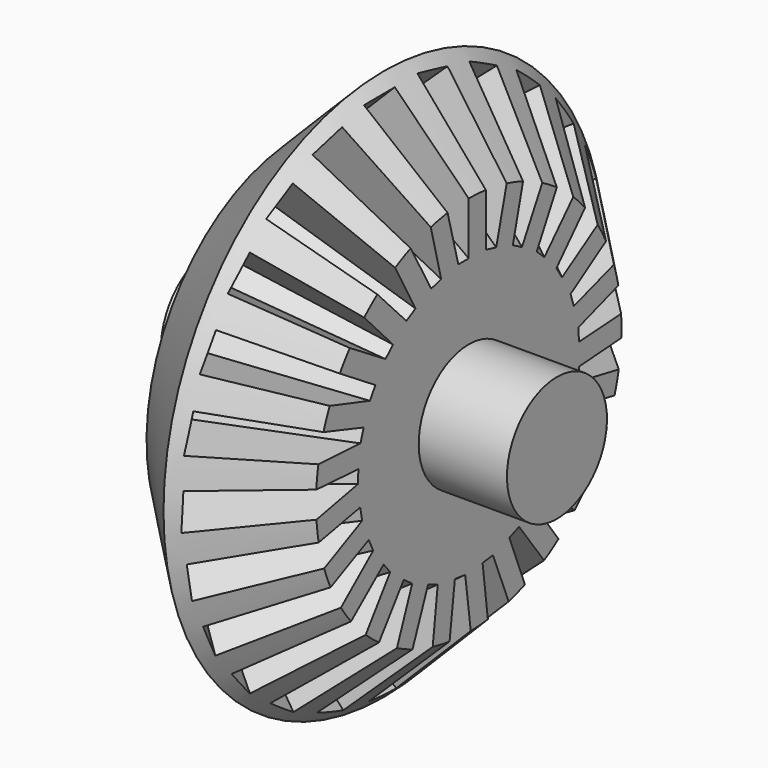
from build123d import *

# Parameters (mm, degrees)
F7_COUNT = 25
F7_ANGLE = 345.6


with BuildPart() as f1:
    # F0 (on Front) → F1 (revolve)
    with BuildSketch(Plane.XZ):
        Polygon((5.5470483679, 18.0012998082), (0.0122273423, 12.4664593884), (-0.0058063755, 4.0821318731), (-5.763291413, 4.0821318731), (-5.763291413, 0), (0, 0), (16.8451661991, 0), (16.8451661991, 4.0821318731), (11.0818887877, 4.0821318731), (11.0818887877, 12.4664787826), align=None)
    revolve(axis=Axis((8.4225830996, 0, 0), (-1, 0, 0)))


with BuildPart() as f6:
    # F5 (on face) → F6 section 0
    with BuildSketch(Plane(origin=(-5.5200079815, 0, 5.5199886393), x_dir=(0, -1, 0), z_dir=(-0.70710802, 0, 0.7071055423)), mode=Mode.PRIVATE) as f6_s0:
        Polygon((0, 16.6512121101), (0, 12.7288497215), (1.3675010996, 12.7288497215), (2.4401100818, 16.6512121101), align=None)
    loft([f6_s0.sketch, Vertex(23.5484112532, 0, 0)])


with BuildPart() as f7_1:
    # F7: instance of F6
    add(f6.part.rotate(Axis((16.8451661991, 0, 0), (-1, 0, 0)), 1 * F7_ANGLE / (F7_COUNT - 1)))


with BuildPart() as f7_2:
    # F7: instance of F6
    add(f6.part.rotate(Axis((16.8451661991, 0, 0), (-1, 0, 0)), 2 * F7_ANGLE / (F7_COUNT - 1)))


with BuildPart() as f7_3:
    # F7: instance of F6
    add(f6.part.rotate(Axis((16.8451661991, 0, 0), (-1, 0, 0)), 3 * F7_ANGLE / (F7_COUNT - 1)))


with BuildPart() as f7_4:
    # F7: instance of F6
    add(f6.part.rotate(Axis((16.8451661991, 0, 0), (-1, 0, 0)), 4 * F7_ANGLE / (F7_COUNT - 1)))


with BuildPart() as f7_5:
    # F7: instance of F6
    add(f6.part.rotate(Axis((16.8451661991, 0, 0), (-1, 0, 0)), 5 * F7_ANGLE / (F7_COUNT - 1)))


with BuildPart() as f7_6:
    # F7: instance of F6
    add(f6.part.rotate(Axis((16.8451661991, 0, 0), (-1, 0, 0)), 6 * F7_ANGLE / (F7_COUNT - 1)))


with BuildPart() as f7_7:
    # F7: instance of F6
    add(f6.part.rotate(Axis((16.8451661991, 0, 0), (-1, 0, 0)), 7 * F7_ANGLE / (F7_COUNT - 1)))


with BuildPart() as f7_8:
    # F7: instance of F6
    add(f6.part.rotate(Axis((16.8451661991, 0, 0), (-1, 0, 0)), 8 * F7_ANGLE / (F7_COUNT - 1)))


with BuildPart() as f7_9:
    # F7: instance of F6
    add(f6.part.rotate(Axis((16.8451661991, 0, 0), (-1, 0, 0)), 9 * F7_ANGLE / (F7_COUNT - 1)))


with BuildPart() as f7_10:
    # F7: instance of F6
    add(f6.part.rotate(Axis((16.8451661991, 0, 0), (-1, 0, 0)), 10 * F7_ANGLE / (F7_COUNT - 1)))


with BuildPart() as f7_11:
    # F7: instance of F6
    add(f6.part.rotate(Axis((16.8451661991, 0, 0), (-1, 0, 0)), 11 * F7_ANGLE / (F7_COUNT - 1)))


with BuildPart() as f7_12:
    # F7: instance of F6
    add(f6.part.rotate(Axis((16.8451661991, 0, 0), (-1, 0, 0)), 12 * F7_ANGLE / (F7_COUNT - 1)))


with BuildPart() as f7_13:
    # F7: instance of F6
    add(f6.part.rotate(Axis((16.8451661991, 0, 0), (-1, 0, 0)), 13 * F7_ANGLE / (F7_COUNT - 1)))


with BuildPart() as f7_14:
    # F7: instance of F6
    add(f6.part.rotate(Axis((16.8451661991, 0, 0), (-1, 0, 0)), 14 * F7_ANGLE / (F7_COUNT - 1)))


with BuildPart() as f7_15:
    # F7: instance of F6
    add(f6.part.rotate(Axis((16.8451661991, 0, 0), (-1, 0, 0)), 15 * F7_ANGLE / (F7_COUNT - 1)))


with BuildPart() as f7_16:
    # F7: instance of F6
    add(f6.part.rotate(Axis((16.8451661991, 0, 0), (-1, 0, 0)), 16 * F7_ANGLE / (F7_COUNT - 1)))


with BuildPart() as f7_17:
    # F7: instance of F6
    add(f6.part.rotate(Axis((16.8451661991, 0, 0), (-1, 0, 0)), 17 * F7_ANGLE / (F7_COUNT - 1)))


with BuildPart() as f7_18:
    # F7: instance of F6
    add(f6.part.rotate(Axis((16.8451661991, 0, 0), (-1, 0, 0)), 18 * F7_ANGLE / (F7_COUNT - 1)))


with BuildPart() as f7_19:
    # F7: instance of F6
    add(f6.part.rotate(Axis((16.8451661991, 0, 0), (-1, 0, 0)), 19 * F7_ANGLE / (F7_COUNT - 1)))


with BuildPart() as f7_20:
    # F7: instance of F6
    add(f6.part.rotate(Axis((16.8451661991, 0, 0), (-1, 0, 0)), 20 * F7_ANGLE / (F7_COUNT - 1)))


with BuildPart() as f7_21:
    # F7: instance of F6
    add(f6.part.rotate(Axis((16.8451661991, 0, 0), (-1, 0, 0)), 21 * F7_ANGLE / (F7_COUNT - 1)))


with BuildPart() as f7_22:
    # F7: instance of F6
    add(f6.part.rotate(Axis((16.8451661991, 0, 0), (-1, 0, 0)), 22 * F7_ANGLE / (F7_COUNT - 1)))


with BuildPart() as f7_23:
    # F7: instance of F6
    add(f6.part.rotate(Axis((16.8451661991, 0, 0), (-1, 0, 0)), 23 * F7_ANGLE / (F7_COUNT - 1)))


with BuildPart() as f7_24:
    # F7: instance of F6
    add(f6.part.rotate(Axis((16.8451661991, 0, 0), (-1, 0, 0)), 24 * F7_ANGLE / (F7_COUNT - 1)))


with BuildPart() as f1_1:
    add(f1.part)

    # F8: cut F6, F7_1, F7_2, F7_3, F7_4, F7_5, F7_6, F7_7, F7_8, F7_9, F7_10, F7_11, F7_12, F7_13, F7_14, F7_15, F7_16, F7_17, F7_18, F7_19, F7_20, F7_21, F7_22, F7_23, F7_24
    add(f6.part, mode=Mode.SUBTRACT)
    add(f7_1.part, mode=Mode.SUBTRACT)
    add(f7_2.part, mode=Mode.SUBTRACT)
    add(f7_3.part, mode=Mode.SUBTRACT)
    add(f7_4.part, mode=Mode.SUBTRACT)
    add(f7_5.part, mode=Mode.SUBTRACT)
    add(f7_6.part, mode=Mode.SUBTRACT)
    add(f7_7.part, mode=Mode.SUBTRACT)
    add(f7_8.part, mode=Mode.SUBTRACT)
    add(f7_9.part, mode=Mode.SUBTRACT)
    add(f7_10.part, mode=Mode.SUBTRACT)
    add(f7_11.part, mode=Mode.SUBTRACT)
    add(f7_12.part, mode=Mode.SUBTRACT)
    add(f7_13.part, mode=Mode.SUBTRACT)
    add(f7_14.part, mode=Mode.SUBTRACT)
    add(f7_15.part, mode=Mode.SUBTRACT)
    add(f7_16.part, mode=Mode.SUBTRACT)
    add(f7_17.part, mode=Mode.SUBTRACT)
    add(f7_18.part, mode=Mode.SUBTRACT)
    add(f7_19.part, mode=Mode.SUBTRACT)
    add(f7_20.part, mode=Mode.SUBTRACT)
    add(f7_21.part, mode=Mode.SUBTRACT)
    add(f7_22.part, mode=Mode.SUBTRACT)
    add(f7_23.part, mode=Mode.SUBTRACT)
    add(f7_24.part, mode=Mode.SUBTRACT)


solid = f1_1.part
